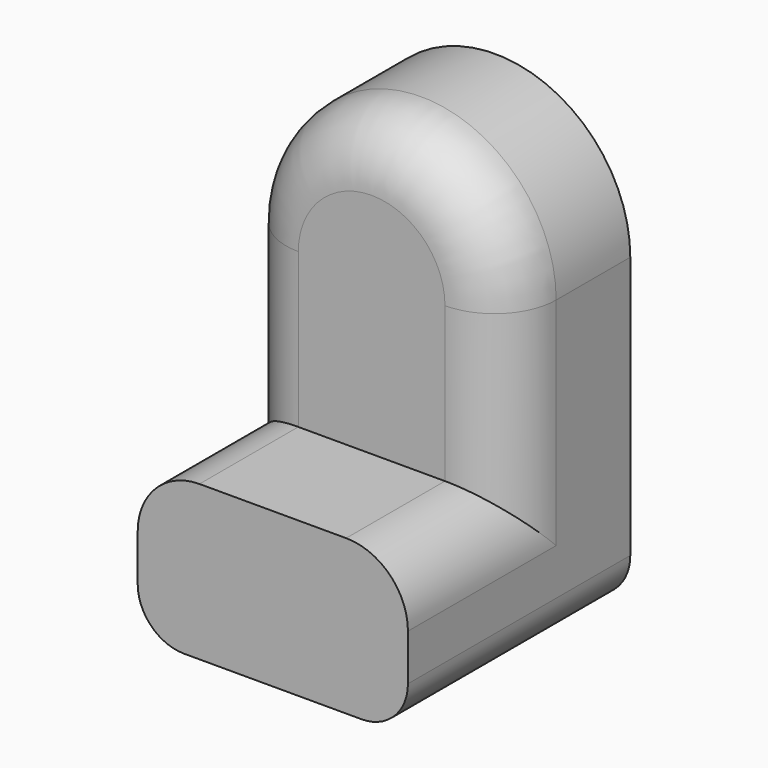
from build123d import *

# Parameters (mm, degrees)
F1_DEPTH = 12.7
F2_W     = 22.225
F2_H     = 12.7
F3_DEPTH = 10.16
F4_R     = 5.08
F5_R     = 3.81
F6_W     = 2.032
F6_H     = 1.016
F7_DEPTH = 1.905
F8_R     = 0.50799


# Not quite as in the source:
# - a fillet or chamfer is up to 0.001 mm smaller than in the source, because OpenCascade refuses the exact size


with BuildPart() as f1:
    # F0 (on Front) → F1 (new body)
    with BuildSketch(Plane.XZ):
        with BuildLine():
            Line((-12.7675240695, 14.3095031442), (-12.7675240695, -11.0904968558))
            Line((-12.7675240695, -11.0904968558), (9.4574759305, -11.0904968558))
            Line((9.4574759305, -11.0904968558), (9.4574759305, 14.3095031442))
            ThreePointArc((9.4574759305, 14.3095031442), (-1.6550240695, 3.1970031442), (-12.7675240695, 14.3095031442))
        make_face()
        with BuildLine():
            ThreePointArc((9.4574759305, 14.3095031442), (-1.6550240695, 25.4220031442), (-12.7675240695, 14.3095031442))
            ThreePointArc((-12.7675240695, 14.3095031442), (-1.6550240695, 3.1970031442), (9.4574759305, 14.3095031442))
        make_face()
    extrude(amount=F1_DEPTH)

    # F2 (on face) → F3 (join)
    with BuildSketch(Plane.XZ.offset(12.7)):
        with Locations((-1.6550240695, -4.7404968558)):
            Rectangle(F2_W, F2_H)
    extrude(amount=F3_DEPTH)

    # F4
    f4_edges = [f1.edges().sort_by_distance(p)[0] for p in [
        (9.457476, -12.7, 7.959503),
        (-12.767524, -17.78, 1.609503),
        (9.457476, -17.78, 1.609503),
    ]]
    fillet(f4_edges, radius=F4_R)

    # F5
    f5_edges = [f1.edges().sort_by_distance(p)[0] for p in [
        (-12.767524, -11.43, -11.090497),
        (9.457476, -11.43, -11.090497),
    ]]
    fillet(f5_edges, radius=F5_R)

    # F6 (on face) → F7 (join)
    with BuildSketch(Plane(origin=(0, 0, 0), x_dir=(-1, 0, 0), z_dir=(0, 1, 0))):
        with Locations((1.6550240695, 14.3095031442)):
            Rectangle(F6_W, F6_H)
    extrude(amount=F7_DEPTH)

    # F8 (radius 0.508 in the source; OpenCascade refuses exactly that, so slightly less here)
    f8_edges = [f1.edges().sort_by_distance(p)[0] for p in [
        (-0.639024, 0.9525, 14.817503),
        (-0.639024, 0.9525, 13.801503),
        (-2.671024, 0.9525, 13.801503),
        (-2.671024, 0.9525, 14.817503),
    ]]
    fillet(f8_edges, radius=F8_R)


solid = f1.part
